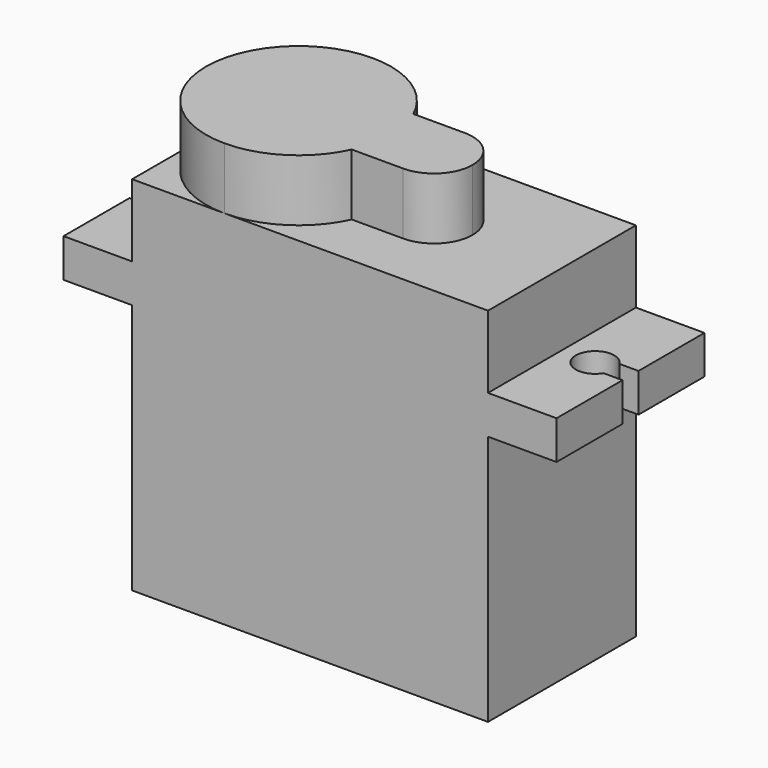
from build123d import *

# Parameters (mm, degrees)
F5_DEPTH = 23.5
F6_START = 16.3
F6_DEPTH = 2.5
F7_DEPTH = 27.5


# Not quite as in the source:
# - ends of sketch curves that miss each other by under 0.0002 mm in the source are joined


with BuildPart() as f5:
    # F4 (on Top) → F5 (new body)
    with BuildSketch(Plane.XY):
        with BuildLine():
            Line((-5.55, -6), (11.55, -6))
            Line((11.55, -6), (11.55, 6))
            Line((11.55, 6), (-5.55, 6))
            ThreePointArc((-5.55, 6), (-2.309629, 5.049752), (-0.095644, 2.5))
            Line((-0.095644, 2.5), (3.24865, 2.5))
            ThreePointArc((3.24865, 2.5), (5.017289, 1.768244), (5.75, 0))
            ThreePointArc((5.75, 0), (5.017289, -1.768244), (3.24865, -2.5))
            Line((3.24865, -2.5), (-0.095644, -2.5))
            ThreePointArc((-0.095644, -2.5), (-2.30963, -5.049753), (-5.55, -6))
        make_face()
        with BuildLine():
            Line((-11.55, 6), (-11.55, 0))
            ThreePointArc((-11.55, 0), (-9.792641, 4.242641), (-5.55, 6))
            Line((-5.55, 6), (-11.55, 6))
        make_face()
        with BuildLine():
            Line((-11.55, -6), (-5.55, -6))
            ThreePointArc((-5.55, -6), (-9.792641, -4.242641), (-11.55, 0))
            Line((-11.55, 0), (-11.55, -6))
        make_face()
        with BuildLine():
            Line((3.24865, 2.5), (3.24865, -2.5))
            ThreePointArc((3.24865, -2.5), (5.017289, -1.768244), (5.75, 0))
            ThreePointArc((5.75, 0), (5.017289, 1.768244), (3.24865, 2.5))
        make_face()
        with BuildLine():
            ThreePointArc((3.24865, 2.5), (0.75, 0), (3.24865, -2.5))
            Line((3.24865, -2.5), (3.24865, 2.5))
        make_face()
        with BuildLine():
            Line((-3.004985, -2.5), (-0.095644, -2.5))
            ThreePointArc((-0.095644, -2.5), (0.312002, -1.279427), (0.45, 0))
            ThreePointArc((0.45, 0), (0.312002, 1.279426), (-0.095644, 2.5))
            Line((-0.095644, 2.5), (-3.004985, 2.5))
            Line((-3.004985, 2.5), (-3.004985, -2.5))
        make_face()
    extrude(amount=F5_DEPTH)



with BuildPart() as f5b:
    # F4 (on Top) → F5, piece 2 (new body)
    with BuildSketch(Plane.XY):
        with BuildLine():
            ThreePointArc((-11.55, 0), (-9.792641, -4.242641), (-5.55, -6))
            ThreePointArc((-5.55, -6), (-2.30963, -5.049753), (-0.095644, -2.5))
            Line((-0.095644, -2.5), (-3.004985, -2.5))
            Line((-3.004985, -2.5), (-3.004985, 2.5))
            Line((-3.004985, 2.5), (-0.095644, 2.5))
            ThreePointArc((-0.095644, 2.5), (-2.309629, 5.049752), (-5.55, 6))
            ThreePointArc((-5.55, 6), (-9.792641, 4.242641), (-11.55, 0))
        make_face()
        with BuildLine():
            ThreePointArc((0.45, 0), (0.312002, -1.279427), (-0.095644, -2.5))
            Line((-0.095644, -2.5), (3.24865, -2.5))
            ThreePointArc((3.24865, -2.5), (0.75, 0), (3.24865, 2.5))
            Line((3.24865, 2.5), (-0.095644, 2.5))
            ThreePointArc((-0.095644, 2.5), (0.312002, 1.279426), (0.45, 0))
        make_face()
    extrude(amount=F5_DEPTH)


with BuildPart() as f5_1:
    add(f5.part)

    add(f5b.part)  # F6 merges F5b
    # F4 (on Top) → F6 (join)
    with BuildSketch(Plane.XY.offset(F6_START)):
        with BuildLine():
            Line((11.55, 6), (11.55, -6))
            Line((11.55, -6), (16, -6))
            Line((16, -6), (16, -0.65))
            Line((16, -0.65), (14.767708, -0.65))
            ThreePointArc((14.767708, -0.65), (12.45, 0), (14.767708, 0.65))
            Line((14.767708, 0.65), (16, 0.65))
            Line((16, 0.65), (16, 6))
            Line((16, 6), (11.55, 6))
        make_face()
        with BuildLine():
            Line((-16, -6), (-11.55, -6))
            Line((-11.55, -6), (-11.55, 0))
            Line((-11.55, 0), (-11.55, 6))
            Line((-11.55, 6), (-16, 6))
            Line((-16, 6), (-16, 0.65))
            Line((-16, 0.65), (-14.767708, 0.65))
            ThreePointArc((-14.767708, 0.65), (-13.362461, 1.203564), (-12.45, 0))
            ThreePointArc((-12.45, 0), (-13.362461, -1.203564), (-14.767708, -0.65))
            Line((-14.767708, -0.65), (-16, -0.65))
            Line((-16, -0.65), (-16, -6))
        make_face()
    extrude(amount=F6_DEPTH)

    # F4 (on Top) → F7 (join)
    with BuildSketch(Plane.XY):
        with BuildLine():
            ThreePointArc((-11.55, 0), (-9.792641, -4.242641), (-5.55, -6))
            ThreePointArc((-5.55, -6), (-2.30963, -5.049753), (-0.095644, -2.5))
            Line((-0.095644, -2.5), (-3.004985, -2.5))
            Line((-3.004985, -2.5), (-3.004985, 2.5))
            Line((-3.004985, 2.5), (-0.095644, 2.5))
            ThreePointArc((-0.095644, 2.5), (-2.309629, 5.049752), (-5.55, 6))
            ThreePointArc((-5.55, 6), (-9.792641, 4.242641), (-11.55, 0))
        make_face()
        with BuildLine():
            Line((-3.004985, -2.5), (-0.095644, -2.5))
            ThreePointArc((-0.095644, -2.5), (0.312002, -1.279427), (0.45, 0))
            ThreePointArc((0.45, 0), (0.312002, 1.279426), (-0.095644, 2.5))
            Line((-0.095644, 2.5), (-3.004985, 2.5))
            Line((-3.004985, 2.5), (-3.004985, -2.5))
        make_face()
        with BuildLine():
            ThreePointArc((0.45, 0), (0.312002, -1.279427), (-0.095644, -2.5))
            Line((-0.095644, -2.5), (3.24865, -2.5))
            ThreePointArc((3.24865, -2.5), (0.75, 0), (3.24865, 2.5))
            Line((3.24865, 2.5), (-0.095644, 2.5))
            ThreePointArc((-0.095644, 2.5), (0.312002, 1.279426), (0.45, 0))
        make_face()
        with BuildLine():
            ThreePointArc((3.24865, 2.5), (0.75, 0), (3.24865, -2.5))
            Line((3.24865, -2.5), (3.24865, 2.5))
        make_face()
        with BuildLine():
            Line((3.24865, 2.5), (3.24865, -2.5))
            ThreePointArc((3.24865, -2.5), (5.017289, -1.768244), (5.75, 0))
            ThreePointArc((5.75, 0), (5.017289, 1.768244), (3.24865, 2.5))
        make_face()
    extrude(amount=F7_DEPTH)


solid = f5_1.part
